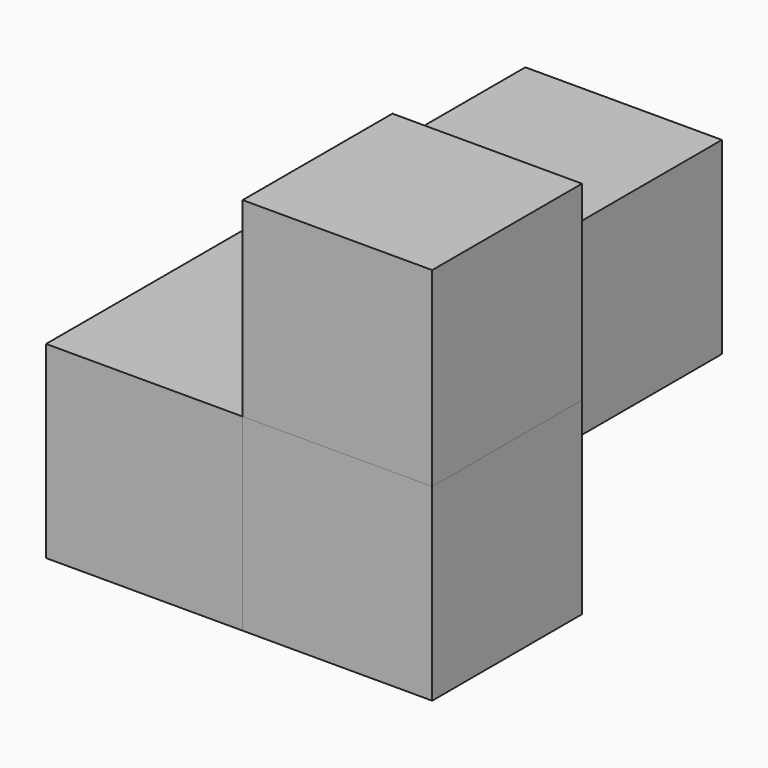
from build123d import *

# Parameters (mm, degrees)
F0_W     = 25.7175005972
F0_H     = 25.8535724133
F1_DEPTH = 25.4
F0_W_2   = 26.6700014472
F0_H_2   = 25.5814287812
F2_DEPTH = 25.4
F3_DEPTH = 25.4
F4_DEPTH = 25.4
F5_DEPTH = 55.88


with BuildPart() as f1:
    # F0 (on Front) → F1 (new body)
    with BuildSketch(Plane.XZ):
        with Locations((-12.8587502986, -12.9267862067)):
            Rectangle(F0_W, F0_H)
    extrude(amount=F1_DEPTH)


with BuildPart() as f2:
    # F0 (on Front) → F2 (new body)
    with BuildSketch(Plane.XZ):
        with Locations((-39.0525013208, -38.6442868039)):
            Rectangle(F0_W_2, F0_H_2)
    extrude(amount=F2_DEPTH)

    # F0 (on Front) → F5 (join)
    with BuildSketch(Plane.XZ):
        with Locations((-39.0525013208, -38.6442868039)):
            Rectangle(F0_W_2, F0_H_2)
    extrude(amount=-F5_DEPTH)


with BuildPart() as f3:
    # F0 (on Front) → F3 (new body)
    with BuildSketch(Plane.XZ):
        with Locations((-12.8587502986, -38.6442868039)):
            Rectangle(F0_W, F0_H_2)
    extrude(amount=F3_DEPTH)


with BuildPart() as f4:
    # F0 (on Front) → F4 (new body)
    with BuildSketch(Plane.XZ):
        with Locations((-12.8587502986, -38.6442868039)):
            Rectangle(F0_W, F0_H_2)
    extrude(amount=F4_DEPTH)


solid = Compound([f1.part, f2.part, f3.part, f4.part])
